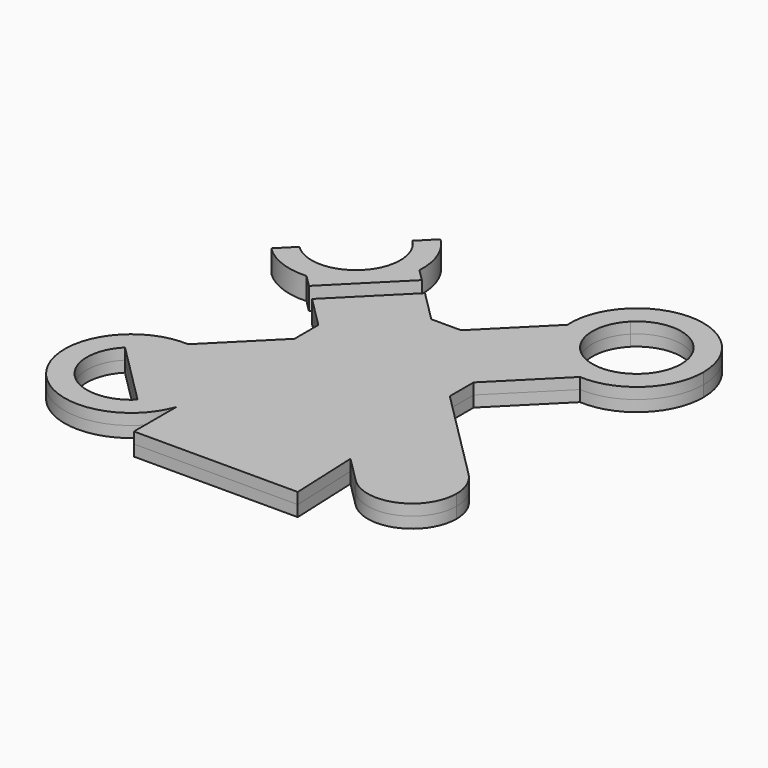
from build123d import *

# Parameters (mm, degrees)
F1_DEPTH = 1


# Not quite as in the source:
# - ends of sketch curves that miss each other by under 0.0002 mm in the source are joined


with BuildPart() as f1:
    # F0 (on Top) → F1 (new body, symmetric)
    with BuildSketch(Plane.XY):
        with BuildLine():
            Line((1.3431457505, 7), (-1.3431457505, 7))
            Line((-1.3431457505, 7), (-4.1715728753, 9.8284271247))
            Line((-4.1715728753, 9.8284271247), (-9.8284271247, 4.1715728753))
            Line((-9.8284271247, 4.1715728753), (-7, 1.3431457505))
            Line((-7, 1.3431457505), (-7, -1.3431457505))
            Line((-7, -1.3431457505), (-7, -12.6568542495))
            Line((-7, -12.6568542495), (-6.6661494646, -12.3230037141))
            Line((-6.6661494646, -12.3230037141), (-1.3431457505, -7))
            Line((-1.3431457505, -7), (1.3431457505, -7))
            Line((1.3431457505, -7), (7.4995861066, -13.1564403561))
            Line((7.4995861066, -13.1564403561), (7, -1.3431457505))
            Line((7, -1.3431457505), (7, 1.3431457505))
            Line((7, 1.3431457505), (12.3230037141, 6.6661494646))
            ThreePointArc((12.3230037141, 6.6661494646), (8.4142135624, 8.4142135624), (6.6661494646, 12.3230037141))
            Line((6.6661494646, 12.3230037141), (1.3431457505, 7))
        make_face()
        with BuildLine():
            ThreePointArc((18.6568542495, 12.6568542495), (12.4898642939, 18.6545299955), (6.6661494646, 12.3230037141))
            Line((6.6661494646, 12.3230037141), (9.8284271247, 15.4852813742))
            ThreePointArc((9.8284271247, 15.4852813742), (14.187587979, 16.3523723795), (16.6568542495, 12.6568542495))
            ThreePointArc((16.6568542495, 12.6568542495), (16.3523723795, 11.12612052), (15.4852813742, 9.8284271247))
            Line((15.4852813742, 9.8284271247), (12.3230037141, 6.6661494646))
            ThreePointArc((12.3230037141, 6.6661494646), (16.7797717109, 8.2977773281), (18.6568542495, 12.6568542495))
        make_face()
        with BuildLine():
            Line((9.8284271247, 15.4852813742), (6.6661494646, 12.3230037141))
            ThreePointArc((6.6661494646, 12.3230037141), (8.4142135624, 8.4142135624), (12.3230037141, 6.6661494646))
            Line((12.3230037141, 6.6661494646), (15.4852813742, 9.8284271247))
            ThreePointArc((15.4852813742, 9.8284271247), (9.8284271247, 9.8284271247), (9.8284271247, 15.4852813742))
        make_face()
        Polygon((-7, -12.6568542495), (-7, -1.3431457505), (-12.3230037141, -6.6661494646), (-15.4852813742, -9.8284271247), (-9.8284271247, -15.4852813742), align=None)
        with BuildLine():
            Line((15.4852813742, -9.8284271247), (7, -1.3431457505))
            Line((7, -1.3431457505), (7.4995861066, -13.1564403561))
            Line((7.4995861066, -13.1564403561), (9.8284271247, -15.4852813742))
            ThreePointArc((9.8284271247, -15.4852813742), (9.8284271247, -9.8284271247), (15.4852813742, -9.8284271247))
        make_face()
        with BuildLine():
            Line((-15.4852813742, -9.8284271247), (-12.3230037141, -6.6661494646))
            ThreePointArc((-12.3230037141, -6.6661494646), (-17.6503476854, -15.9832672282), (-7, -14.6568542495))
            Line((-7, -14.6568542495), (-7, -12.6568542495))
            Line((-7, -12.6568542495), (-9.8284271247, -15.4852813742))
            ThreePointArc((-9.8284271247, -15.4852813742), (-15.4852813742, -15.4852813742), (-15.4852813742, -9.8284271247))
        make_face()
        with BuildLine():
            Line((-6.6661494646, -12.3230037141), (-7, -12.6568542495))
            Line((-7, -12.6568542495), (-7, -14.6568542495))
            ThreePointArc((-7, -14.6568542495), (-6.717315341, -13.5064880262), (-6.6661494646, -12.3230037141))
        make_face()
        with BuildLine():
            ThreePointArc((16.6568542495, -12.6568542495), (16.3523723795, -11.12612052), (15.4852813742, -9.8284271247))
            Line((15.4852813742, -9.8284271247), (9.8284271247, -15.4852813742))
            ThreePointArc((9.8284271247, -15.4852813742), (14.187587979, -16.3523723795), (16.6568542495, -12.6568542495))
        make_face()
        with BuildLine():
            Line((9.8284271247, -15.4852813742), (15.4852813742, -9.8284271247))
            ThreePointArc((15.4852813742, -9.8284271247), (9.8284271247, -9.8284271247), (9.8284271247, -15.4852813742))
        make_face()
        with BuildLine():
            Line((7.7648614533, -19.4291844964), (7.4995861066, -13.1564403561))
            Line((7.4995861066, -13.1564403561), (1.3431457505, -7))
            Line((1.3431457505, -7), (-1.3431457505, -7))
            Line((-1.3431457505, -7), (-6.6661494646, -12.3230037141))
            ThreePointArc((-6.6661494646, -12.3230037141), (-6.717315341, -13.5064880262), (-7, -14.6568542495))
            Line((-7, -14.6568542495), (-7, -19.4291844964))
            Line((-7, -19.4291844964), (7.7648614533, -19.4291844964))
        make_face()
    extrude(amount=F1_DEPTH, both=True)


with BuildPart() as f1b:
    # F0 (on Top) → F1, piece 2 (new body, symmetric)
    with BuildSketch(Plane.XY):
        with BuildLine():
            Line((-5.5857864376, 11.2426406871), (-6.6661494646, 12.3230037141))
            ThreePointArc((-6.6661494646, 12.3230037141), (-7.059654803, 14.8181867913), (-8.4452303219, 16.9302865811))
            Line((-8.4452303219, 16.9302865811), (-9.8529299986, 15.5095737932))
            ThreePointArc((-9.8529299986, 15.5095737932), (-9.8154440182, 9.841470102), (-15.483652679, 9.8267993668))
            Line((-15.483652679, 9.8267993668), (-16.8913523576, 8.4060865808))
            ThreePointArc((-16.8913523576, 8.4060865808), (-14.7924122945, 7.0497701734), (-12.3230037141, 6.6661494646))
            Line((-12.3230037141, 6.6661494646), (-11.2426406871, 5.5857864376))
            Line((-11.2426406871, 5.5857864376), (-5.5857864376, 11.2426406871))
        make_face()
    extrude(amount=F1_DEPTH, both=True)


solid = Compound([f1.part, f1b.part])
